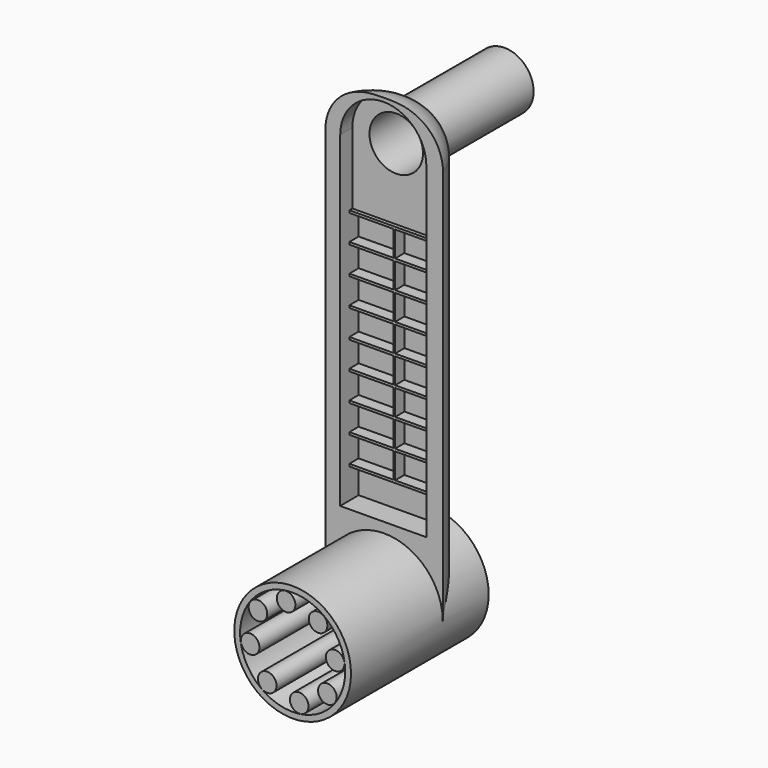
from build123d import *

# Parameters (mm, degrees)
F0_R        = 12.55
F1_DEPTH    = 37
F2_R        = 7.5
F3_DEPTH    = 3
F6_DEPTH    = 95
F7_T2_ANGLE = 359.64
F9_R        = 6.25
F10_DEPTH   = 30
F11_W       = 18.3796742931
F11_H       = 70.2870060131
F12_DEPTH   = 2
F13_DEPTH   = 2.5
F14_W       = 9.4460686669
F14_H       = 6.4466400072
F14_H_2     = 5.4794391096
F14_W_2     = 8.6165779212
F14_W_3     = 0.317027705
F15_DEPTH   = 2.5
F16_DEPTH   = 0.8
F17_R       = 5.7074191609
F18_DEPTH   = 28
F19_R       = 11.3
F20_DEPTH   = 32.8
F21_R       = 2
F22_DEPTH   = 32.8


# Not quite as in the source:
# - a fillet or chamfer that OpenCascade refuses, or shapes differently, is made with other operations: its cross-section is extruded or revolved along the edge and cut away or added


with BuildPart() as f1:
    # F0 (on Front) → F1 (new body)
    with BuildSketch(Plane.XZ):
        Circle(F0_R)
    extrude(amount=F1_DEPTH)

    # F2 (on Front) → F3 (join)
    with BuildSketch(Plane.XZ):
        Circle(F2_R)
    extrude(amount=-F3_DEPTH)

    # F4: fillet of radius 10 on 1 edges, made by hand

    # F4_s1 → F4_t2 (revolve, cut)
    with BuildSketch(Plane.XY):
        with BuildLine():
            ThreePointArc((7.5, 0), (4.2315549177, 2.2195444573), (0.3585715715, 3))
            Line((0.3585715715, 3), (7.5, 3))
            Line((7.5, 3), (7.5, 0))
        make_face()
    revolve(axis=Axis((0, 3, 0), (0, -1, 0)), mode=Mode.SUBTRACT)

    # F5 (on Top) → F6 (join)
    with BuildSketch(Plane.XY):
        with BuildLine():
            Line((-12.4928209826, -12.5774559094), (12.6060726016, -12.3417848491))
            ThreePointArc((12.6060726016, -12.3417848491), (-0.0335977446, -2.8508403226), (-12.4928209826, -12.5774559094))
        make_face()
    extrude(amount=F6_DEPTH)

    # F7: fillet of radius 10 on 1 edges, made by hand

    # F7_s1 → F7_t2 (revolve, cut)
    with BuildSketch(Plane(origin=(-0.1101500857, -0.0013803647, 0), x_dir=(0, 0, 1), z_dir=(-0.9999214878, -0.0125306879, 0))):
        with BuildLine():
            ThreePointArc((85, -28.8501313418), (92.0710678119, -25.9211991536), (95, -18.8501313418))
            Line((95, -18.8501313418), (95, -28.8501313418))
            Line((95, -28.8501313418), (85, -28.8501313418))
        make_face()
    revolve(axis=Axis((0.0884629639, -15.8502672786, 95), (0, 0, 1)), revolution_arc=F7_T2_ANGLE, mode=Mode.SUBTRACT)

    # F9 (on offset) → F10 (join)
    with BuildSketch(Plane.XZ.offset(10)):
        with Locations((-0.0335977446, 85)):
            Circle(F9_R)
    extrude(amount=-F10_DEPTH)

    # F11 (on face) → F12 (cut)
    with BuildSketch(Plane(origin=(0.1169867653, -12.4590536081, 0), x_dir=(0.9999559197, 0.0093892853, 0), z_dir=(0.0093892853, -0.9999559197, 0))):
        with Locations((-0.2562315203, 49.8564969935)):
            Rectangle(F11_W, F11_H)
    extrude(amount=-F12_DEPTH, mode=Mode.SUBTRACT)

    # F11 (on face) → F13 (cut)
    with BuildSketch(Plane(origin=(0.1169867653, -12.4590536081, 0), x_dir=(0.9999559197, 0.0093892853, 0), z_dir=(0.0093892853, -0.9999559197, 0))):
        with BuildLine():
            ThreePointArc((8.9336056262, 85), (-0.2562315203, 94.1898371466), (-9.4460686669, 85))
            Line((-9.4460686669, 85), (8.9336056262, 85))
        make_face()
        with Locations((-0.2562315203, 49.8564969935)):
            Rectangle(F11_W, F11_H)
    extrude(amount=-F13_DEPTH, mode=Mode.SUBTRACT)

    # F14 (on face) → F15 (cut)
    with BuildSketch(Plane(origin=(0.0935135522, -9.9591638088, 0), x_dir=(0.9999559197, 0.0093892853, 0), z_dir=(0.0093892853, -0.9999559197, 0))):
        with Locations((-4.7230343334, 17.9363139905)):
            Rectangle(F14_W, F14_H)
        with Locations((-4.7230343334, 24.4199144393)):
            Rectangle(F14_W, F14_H_2)
        with Locations((-4.7230343334, 30.4199144393)):
            Rectangle(F14_W, F14_H_2)
        with Locations((-4.7230343334, 36.4199144393)):
            Rectangle(F14_W, F14_H_2)
        with Locations((-4.7230343334, 42.4199144393)):
            Rectangle(F14_W, F14_H_2)
        with Locations((-4.7230343334, 48.4199144393)):
            Rectangle(F14_W, F14_H_2)
        with Locations((-4.7230343334, 54.4199144393)):
            Rectangle(F14_W, F14_H_2)
        with Locations((-4.7230343334, 60.4199144393)):
            Rectangle(F14_W, F14_H_2)
        with Locations((-4.7230343334, 66.4199144393)):
            Rectangle(F14_W, F14_H_2)
        with Locations((4.6253166656, 66.4199144393)):
            Rectangle(F14_W_2, F14_H_2)
        with Locations((4.6253166656, 60.4199144393)):
            Rectangle(F14_W_2, F14_H_2)
        with Locations((4.6253166656, 54.4199144393)):
            Rectangle(F14_W_2, F14_H_2)
        with Locations((4.6253166656, 48.4199144393)):
            Rectangle(F14_W_2, F14_H_2)
        with Locations((4.6253166656, 42.4199144393)):
            Rectangle(F14_W_2, F14_H_2)
        with Locations((4.6253166656, 36.4199144393)):
            Rectangle(F14_W_2, F14_H_2)
        with Locations((4.6253166656, 30.4199144393)):
            Rectangle(F14_W_2, F14_H_2)
        with Locations((4.6253166656, 24.4199144393)):
            Rectangle(F14_W_2, F14_H_2)
        with Locations((0.1585138525, 17.9363139905)):
            Rectangle(F14_W_3, F14_H)
        with Locations((4.6253166656, 17.9363139905)):
            Rectangle(F14_W_2, F14_H)
    extrude(amount=-F15_DEPTH, mode=Mode.SUBTRACT)

    # F14 (on face) → F16 (cut)
    with BuildSketch(Plane(origin=(0.0935135522, -9.9591638088, 0), x_dir=(0.9999559197, 0.0093892853, 0), z_dir=(0.0093892853, -0.9999559197, 0))):
        with BuildLine():
            Line((-9.4460686669, 85), (-9.4460686669, 69.6801948845))
            Line((-9.4460686669, 69.6801948845), (0, 69.6801948845))
            Line((0, 69.6801948845), (0.317027705, 69.6801948845))
            Line((0.317027705, 69.6801948845), (8.9336056262, 69.6801948845))
            Line((8.9336056262, 69.6801948845), (8.9336056262, 85))
            ThreePointArc((8.9336056262, 85), (-0.2562315203, 94.1898371466), (-9.4460686669, 85))
        make_face()
    extrude(amount=-F16_DEPTH, mode=Mode.SUBTRACT)

    # F17 (on face) → F18 (cut)
    with BuildSketch(Plane.XZ.offset(10)):
        with Locations((0, 84.9810764194)):
            Circle(F17_R)
    extrude(amount=-F18_DEPTH, mode=Mode.SUBTRACT)

    # F19 (on face) → F20 (cut)
    with BuildSketch(Plane.XZ.offset(37)):
        Circle(F19_R)
    extrude(amount=-F20_DEPTH, mode=Mode.SUBTRACT)

    # F21 (on face) → F22 (join)
    with BuildSketch(Plane.XZ.offset(4.2)):
        with Locations((-7.4610639253, 5.4676343242)):
            Circle(F21_R)
        with Locations((-9.1419702041, -1.4095675888)):
            Circle(F21_R)
        with Locations((-5.4676343242, -7.4610639253)):
            Circle(F21_R)
        with Locations((1.4095675888, -9.1419702041)):
            Circle(F21_R)
        with Locations((7.4610639253, -5.4676343242)):
            Circle(F21_R)
        with Locations((9.1419702041, 1.4095675888)):
            Circle(F21_R)
        with Locations((5.4676343242, 7.4610639253)):
            Circle(F21_R)
        with Locations((-1.4095675888, 9.1419702041)):
            Circle(F21_R)
    extrude(amount=F22_DEPTH)


solid = f1.part
